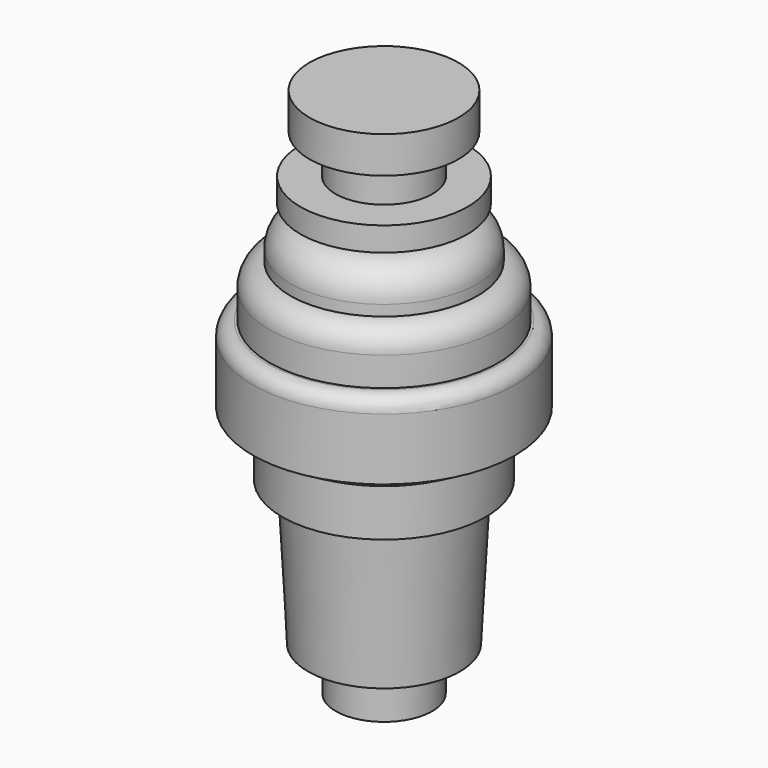
from build123d import *

# Parameters (mm, degrees)
F2_R = 25.7548302834
F4_R = 11.650994652


# Not quite as in the source:
# - a fillet or chamfer that OpenCascade refuses, or shapes differently, is made with other operations: its cross-section is extruded or revolved along the edge and cut away or added


with BuildPart() as f1:
    # F0 (on Front) → F1 (revolve)
    with BuildSketch(Plane.XZ):
        Polygon((0, 0), (0, 437.0113793103), (-61.3251142204, 437.0113793103), (-61.3251142204, 406.9045186043), (-39.9097763002, 406.9045186043), (-39.9097763002, 374.7815191746), (-68.7381178141, 374.7815191746), (-68.7381178141, 355.0135195255), (-48.9701107144, 355.0135195255), (-48.9701107144, 347.6004898548), (-76.974786818, 347.6004898548), (-76.974786818, 313.006490469), (-94.2717939615, 313.006490469), (-94.2717939615, 270.1758146286), (-107.95, 270.1758146286), (-107.95, 207.5771391392), (-83.5641175508, 193.5748010874), (-83.5641175508, 154.8624634743), (-68.7381178141, 154.8624634743), (-62.401818486, 36.0568519682), (-39.6875, 36.0568519682), (-39.6875, 0), align=None)
    revolve(axis=Axis((0, 0, 218.5056896552), (0, 0, -1)))

    # F2
    f2_edges = [f1.edges().sort_by_distance(p)[0] for p in [
        (76.974787, 0, 347.60049),
    ]]
    fillet(f2_edges, radius=F2_R)

    # F3: fillet of radius 19.0095175901 on 1 edges, made by hand

    # F3_s1 → F3_t2 (revolve, cut)
    with BuildSketch(Plane.XZ):
        with BuildLine():
            ThreePointArc((-76.974786818, 313.006490469), (-89.296444613, 306.8962751619), (-94.2717939615, 294.0742674886))
            Line((-94.2717939615, 294.0742674886), (-94.2717939615, 313.006490469))
            Line((-94.2717939615, 313.006490469), (-76.974786818, 313.006490469))
        make_face()
    revolve(axis=Axis((0, 0, 313.006490469), (0, 0, -1)), mode=Mode.SUBTRACT)

    # F4
    f4_edges = [f1.edges().sort_by_distance(p)[0] for p in [
        (107.95, 0, 270.175815),
    ]]
    fillet(f4_edges, radius=F4_R)


solid = f1.part
